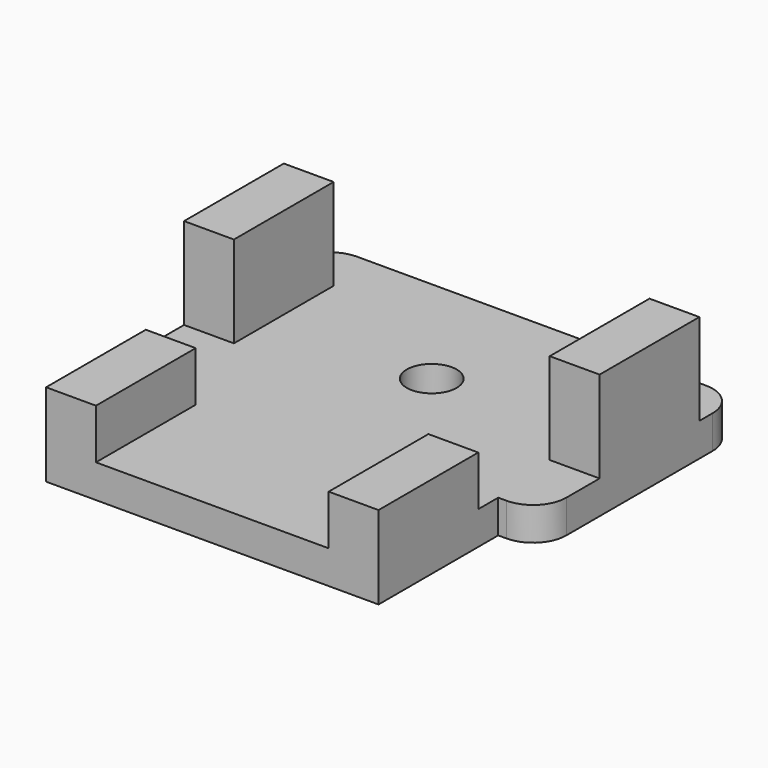
from build123d import *

# Parameters (mm, degrees)
F0_R     = 1.5
F1_DEPTH = 2
F2_W     = 3
F2_H     = 7.5
F3_DEPTH = 3
F4_DEPTH = 5.5
F5_R     = 2


# Not quite as in the source:
# - a pattern or mirror of a feature is missing from the dataset's text; its kind, count and spacing are read off the source's solid


with BuildPart() as f1:
    # F0 (on Top) → F1 (new body)
    with BuildSketch(Plane.XY):
        Polygon((12.5, 12), (0, 12), (-12.5, 12), (-12.5, -3), (-10, -3), (-10, -12), (0, -12), (10, -12), (10, -3), (12.5, -3), align=None)
        with Locations((0, 4.5)):
            Circle(F0_R, mode=Mode.SUBTRACT)
    extrude(amount=F1_DEPTH)

    # F2 (on face) → F3 (join)
    with BuildSketch(Plane.XY.offset(2)):
        with Locations((8.5, -8.25)):
            Rectangle(F2_W, F2_H)
    f3 = extrude(amount=F3_DEPTH)

    # F3_copies: F3 across plane
    add(f3.mirror(Plane(origin=(0, 0, 0), x_dir=(0, 0, -1), z_dir=(-1, 0, 0))))

    # F2 (on face) → F4 (join)
    with BuildSketch(Plane.XY.offset(2)):
        with Locations((11, 5.25)):
            Rectangle(F2_W, F2_H)
    f4 = extrude(amount=F4_DEPTH)

    # F4_copies: F4 across plane
    add(f4.mirror(Plane(origin=(0, 0, 0), x_dir=(0, 0, -1), z_dir=(-1, 0, 0))))

    # F5
    f5_edges = [f1.edges().sort_by_distance(p)[0] for p in [
        (12.5, 12, 1),
        (12.5, -3, 1),
        (-12.5, -3, 1),
        (-12.5, 12, 1),
    ]]
    fillet(f5_edges, radius=F5_R)


solid = f1.part
